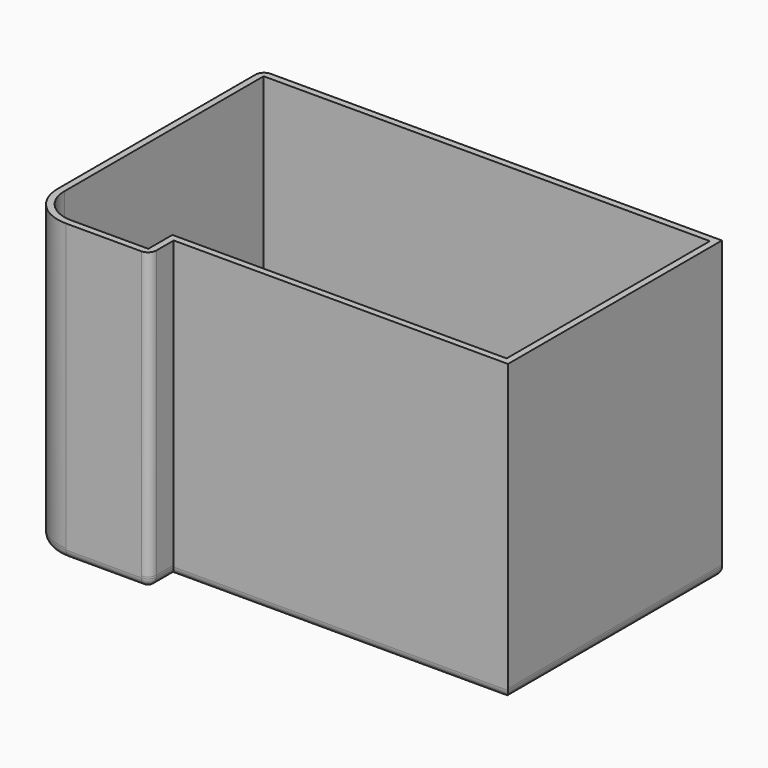
from build123d import *

# Parameters (mm, degrees)
F1_DEPTH     = 1.524
F3_DEPTH     = 43.434
F4_R         = 1.27
F5_T1_DEPTH  = 0.254
F5_T3_DEPTH  = 46.609
F5_S7_W      = 1.27
F5_S7_H      = 1.27
F5_T8_DEPTH  = 1.27
F5_S13_W     = 1.27
F5_S13_H     = 1.27
F5_T14_DEPTH = 1.27


# Not quite as in the source:
# - a fillet or chamfer that OpenCascade refuses, or shapes differently, is made with other operations: its cross-section is extruded or revolved along the edge and cut away or added


with BuildPart() as f1:
    # F0 (on Top) → F1 (new body)
    with BuildSketch(Plane.XY):
        with BuildLine():
            Line((-35.579891, 21.538353), (-35.579891, -17.323647))
            ThreePointArc((-35.579891, -17.323647), (-33.720019, -21.813775), (-29.229891, -23.673647))
            Line((-29.229891, -23.673647), (-16.529891, -23.673647))
            Line((-16.529891, -23.673647), (-16.529891, -19.101647))
            Line((-16.529891, -19.101647), (34.270109, -19.101647))
            Line((34.270109, -19.101647), (34.270109, 21.538353))
            Line((34.270109, 21.538353), (-35.579891, 21.538353))
        make_face()
    extrude(amount=F1_DEPTH)

    # F2 (on face) → F3 (join)
    with BuildSketch(Plane.XY.offset(1.524)):
        with BuildLine():
            Line((-35.57989, 21.538353), (-35.57989, -17.323647))
            ThreePointArc((-35.57989, -17.323647), (-33.720018, -21.813775), (-29.22989, -23.673647))
            Line((-29.22989, -23.673647), (-16.52989, -23.673647))
            Line((-16.52989, -23.673647), (-16.52989, -19.101647))
            Line((-16.52989, -19.101647), (34.27011, -19.101647))
            Line((34.27011, -19.101647), (34.27011, 21.538353))
            Line((34.27011, 21.538353), (-35.57989, 21.538353))
        make_face()
        with BuildLine():
            Line((33.25411, -18.085647), (-17.54589, -18.085647))
            Line((-17.54589, -18.085647), (-17.54589, -22.657647))
            Line((-17.54589, -22.657647), (-29.22989, -22.657647))
            ThreePointArc((-29.22989, -22.657647), (-33.001598, -21.095355), (-34.56389, -17.323647))
            Line((-34.56389, -17.323647), (-34.56389, 20.522353))
            Line((-34.56389, 20.522353), (33.25411, 20.522353))
            Line((33.25411, 20.522353), (33.25411, -18.085647))
        make_face(mode=Mode.SUBTRACT)
    extrude(amount=F3_DEPTH)

    # F4
    f4_edges = [f1.edges().sort_by_distance(p)[0] for p in [
        (-0.654891, 21.538353, 0),
        (-35.579891, 2.107353, 0),
        (-33.720019, -21.813775, 0),
        (-22.879891, -23.673647, 0),
        (-16.529891, -21.387647, 0),
        (8.870109, -19.101647, 0),
        (34.270109, 1.218353, 0),
    ]]
    fillet(f4_edges, radius=F4_R)

    # F5: fillet of radius 1.27 on 4 edges, made by hand

    # F5_s2 → F5_t1 (cut)
    with BuildSketch(Plane.XY.offset(1.27)):
        with BuildLine():
            ThreePointArc((-17.799891, -23.673647), (-16.901866, -23.301673), (-16.529891, -22.403647))
            Line((-16.529891, -22.403647), (-16.529891, -23.673647))
            Line((-16.529891, -23.673647), (-17.799891, -23.673647))
        make_face()
        with BuildLine():
            ThreePointArc((-34.309891, 21.538353), (-35.207917, 21.166379), (-35.579891, 20.268353))
            Line((-35.579891, 20.268353), (-35.579891, 21.538353))
            Line((-35.579891, 21.538353), (-34.309891, 21.538353))
        make_face()
    extrude(amount=F5_T1_DEPTH, mode=Mode.SUBTRACT)

    # F5_s4 → F5_t3 (cut)
    with BuildSketch(Plane.XY.offset(1.524)):
        with BuildLine():
            ThreePointArc((-17.79989, -23.673647), (-16.901864, -23.301673), (-16.52989, -22.403647))
            Line((-16.52989, -22.403647), (-16.52989, -23.673647))
            Line((-16.52989, -23.673647), (-17.79989, -23.673647))
        make_face()
        with BuildLine():
            ThreePointArc((-34.30989, 21.538353), (-35.207916, 21.166379), (-35.57989, 20.268353))
            Line((-35.57989, 20.268353), (-35.57989, 21.538353))
            Line((-35.57989, 21.538353), (-34.30989, 21.538353))
        make_face()
    extrude(amount=F5_T3_DEPTH, mode=Mode.SUBTRACT)


with BuildPart() as f5_tool6:
    # F5_s7 → F5_t8 (new body)
    with BuildSketch(Plane.XZ.offset(-20.268353)):
        with Locations((-34.944891, 0.635)):
            Rectangle(F5_S7_W, F5_S7_H)
    extrude(amount=-F5_T8_DEPTH)

    # F5_s9 → F5_t10 (revolve, cut)
    with BuildSketch(Plane(origin=(-34.309891, 20.268353, 1.27), x_dir=(0.707107, 0, 0.707107), z_dir=(-0.707107, 0, 0.707107))):
        with BuildLine():
            ThreePointArc((0, -1.27), (1.27, 0), (0, 1.27))
            Line((0, 1.27), (0, -1.27))
        make_face()
    revolve(axis=Axis((-34.309891, 20.268353, 1.27), (0, 1, 0)), mode=Mode.SUBTRACT)


with BuildPart() as f1_1:
    add(f1.part)

    # F5_t5: cut F5_tool6
    add(f5_tool6.part, mode=Mode.SUBTRACT)


with BuildPart() as f5_tool12:
    # F5_s13 → F5_t14 (new body)
    with BuildSketch(Plane.XZ.offset(22.403647)):
        with Locations((-17.164891, 0.635)):
            Rectangle(F5_S13_W, F5_S13_H)
    extrude(amount=F5_T14_DEPTH)

    # F5_s15 → F5_t16 (revolve, cut)
    with BuildSketch(Plane(origin=(-17.799891, -22.403647, 1.27), x_dir=(-0.707107, 0, 0.707107), z_dir=(0.707107, 0, 0.707107))):
        with BuildLine():
            ThreePointArc((0, -1.27), (1.27, 0), (0, 1.27))
            Line((0, 1.27), (0, -1.27))
        make_face()
    revolve(axis=Axis((-17.799891, -22.403647, 1.27), (0, -1, 0)), mode=Mode.SUBTRACT)


with BuildPart() as f1_2:
    add(f1_1.part)

    # F5_t11: cut F5_tool12
    add(f5_tool12.part, mode=Mode.SUBTRACT)


solid = f1_2.part
